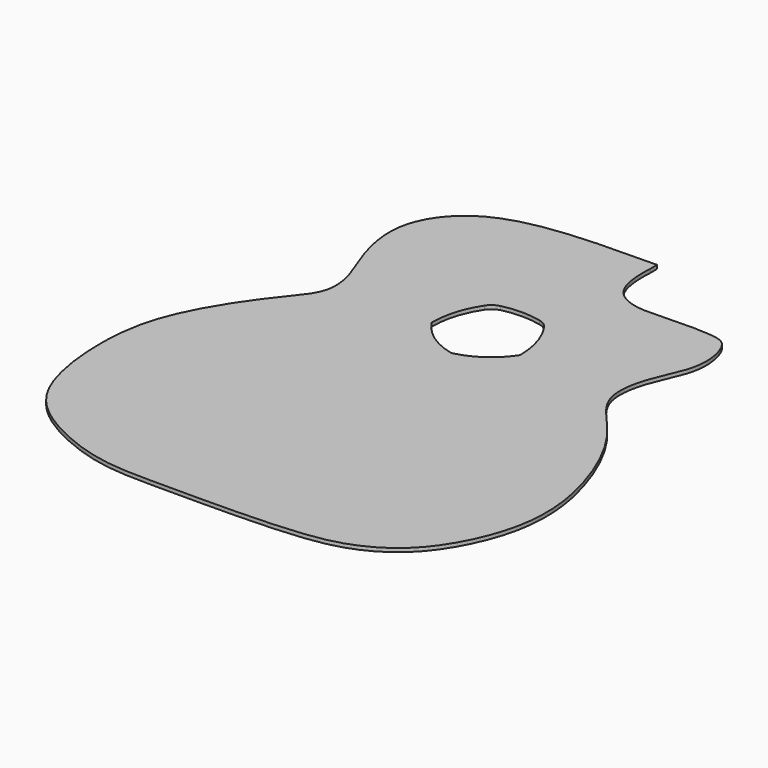
from build123d import *

# Parameters (mm, degrees)
F2_DEPTH = 3.175
F3_DEPTH = 25.4


# Not quite as in the source:
# - a length typed as a fraction of an inch, garbled in the dataset ("3 / 203.2 mm" for 3/8 in), is restored


with BuildPart() as f2:
    # F1 (on Top) → F2 (new body)
    with BuildSketch(Plane.XY):
        with BuildLine():
            Line((27.9880836606, 144.9291706085), (27.9880836606, 152.4919718504))
            add(Edge.make_bspline(
                [(27.9880836606, 152.4919718504), (-21.2502434403, 151.9818123943), (-104.683480426, 152.5111781702), (-150.2814387338, 92.5478236213), (-136.3499609731, 37.8358402777), (-123.192038006, 10.5203140923), (-120.0692970968, -19.2419116422), (-145.6437445747, -45.8599929551), (-184.1291247278, -104.1883013851), (-196.0881801563, -159.8505304336), (-190.1024130042, -227.3864691226), (-165.1049172353, -273.8463464795), (-94.3572995114, -306.4869610902), (-36.2892985312, -306.3059086721), (84.6805760335, -306.6141635236), (130.6656399599, -293.9057736233), (167.9098450774, -267.8044247049), (198.4433715448, -205.4720909521), (195.0092388083, -136.4120768934), (162.1262885831, -60.2938889287), (118.4914998889, -24.7927772039), (126.0312180506, 20.2608585453), (145.9616839168, 53.9116622232), (138.3139785197, 88.5841734777), (124.0639874193, 97.2876685095), (76.6307897746, 95.335485595), (53.1700687674, 94.6735408278), (31.6095759071, 105.7118995447), (27.2876604892, 130.3849807454), (27.7738659058, 140.4809686851), (27.9880836606, 144.9291706085)],
                knots=[0, 0, 0, 0, 0.0589504135, 0.0992297739, 0.1362515931, 0.164817668, 0.1908938507, 0.221359958, 0.2640625563, 0.303291658, 0.3447276857, 0.3814034425, 0.4246551727, 0.4654184817, 0.5214407122, 0.5569335895, 0.5901784057, 0.6318735276, 0.6746616904, 0.7211462663, 0.7581591041, 0.7905331897, 0.8229808841, 0.851507782, 0.8712985789, 0.9062296252, 0.9319829029, 0.9555647239, 0.9804182413, 1, 1, 1, 1], degree=3))
        make_face()
    extrude(amount=-F2_DEPTH)

    # F0 (on Top) → F3 (cut)
    with BuildSketch(Plane.XY):
        with BuildLine():
            ThreePointArc((-16.8686046723, 39.694722813), (-21.8296031184, 37.4568004538), (-25.6371865623, 33.5680846779))
            ThreePointArc((-25.6371865623, 33.5680846779), (-34.9158052402, 13.9395799822), (-38.1, -7.5367294048))
            ThreePointArc((-38.1, -7.5367294048), (-38.0061008622, -8.1700471152), (-37.7324824564, -8.7488746701))
            ThreePointArc((-37.7324824564, -8.7488746701), (-21.8138558814, -25.0066967788), (-1.0730676971, -34.3629330545))
            ThreePointArc((-1.0730676971, -34.3629330545), (0, -34.4910638238), (1.0730676971, -34.3629330545))
            ThreePointArc((1.0730676971, -34.3629330545), (21.8138558814, -25.0066967788), (37.7324824564, -8.7488746701))
            ThreePointArc((37.7324824564, -8.7488746701), (38.0061008622, -8.1700471152), (38.1, -7.5367294048))
            ThreePointArc((38.1, -7.5367294048), (34.9158052402, 13.9395799822), (25.6371865623, 33.5680846779))
            ThreePointArc((25.6371865623, 33.5680846779), (21.8296031184, 37.4568004538), (16.8686046723, 39.694722813))
            ThreePointArc((16.8686046723, 39.694722813), (0, 41.7089361762), (-16.8686046723, 39.694722813))
        make_face()
    extrude(amount=-F3_DEPTH, mode=Mode.SUBTRACT)


solid = f2.part
